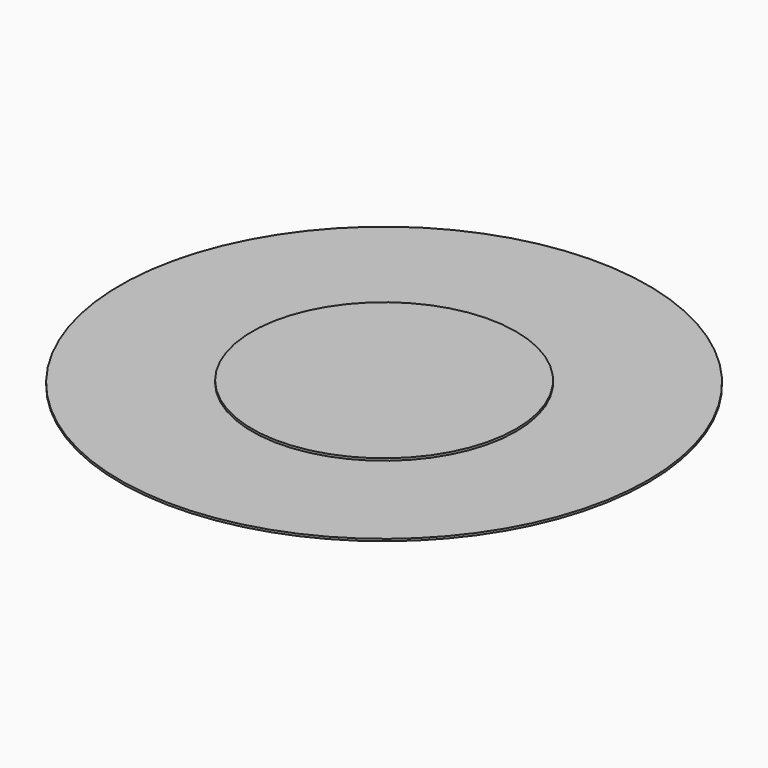
from build123d import *

# Parameters (mm, degrees)
F0_R     = 25
F1_DEPTH = 0.2
F2_R     = 12.5
F3_DEPTH = 0.21


with BuildPart() as f1:
    # F0 (on Top) → F1 (new body)
    with BuildSketch(Plane.XY):
        Circle(F0_R)
    extrude(amount=F1_DEPTH)

    # F2 (on face) → F3 (join)
    with BuildSketch(Plane.XY.offset(0.2)):
        Circle(F2_R)
    extrude(amount=F3_DEPTH)


solid = f1.part
